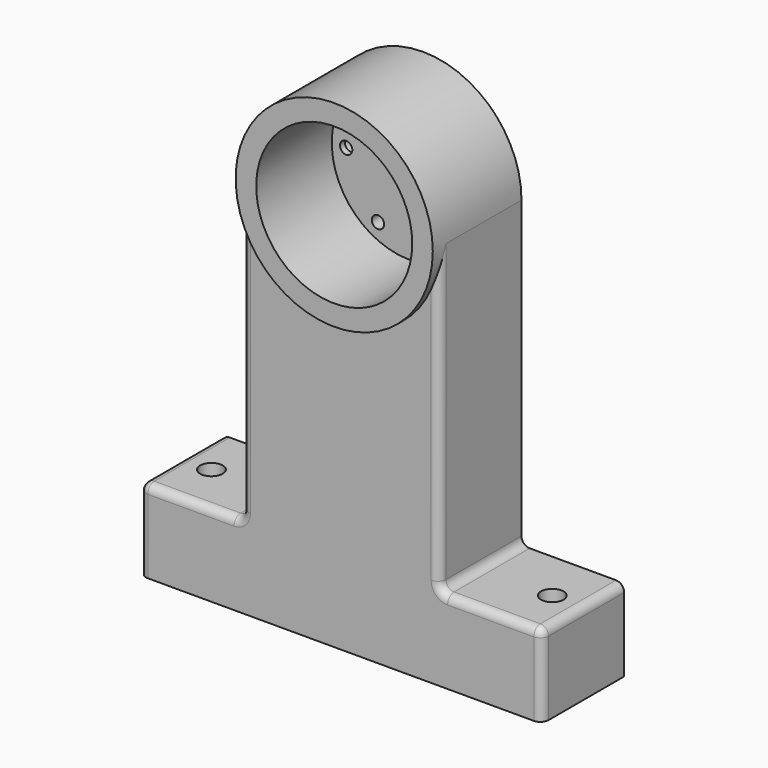
from build123d import *

# Parameters (mm, degrees)
F0_R          = 19
F0_R_2        = 1.5
F0_R_3        = 6.1
F1_DEPTH      = 4
F2_R          = 24
F2_R_2        = 19
F3_DEPTH      = 27
F5_DEPTH      = 25
F6_R          = 2.65
F7_DEPTH      = 2.5
F8_W          = 24
F8_H          = 54
F9_DEPTH      = 25
F10_W         = 25
F10_H         = 20
F11_DEPTH     = 25
F13_W         = 25
F13_H         = 20
F14_DEPTH     = 25
F15_R         = 2
F17_DEPTH     = 25
F18_DEPTH     = 25
F19_T1_DEPTH  = 25
F19_T3_DEPTH  = 21
F19_T5_DEPTH  = 23
F19_T7_DEPTH  = 21
F19_T12_DEPTH = 87
F19_S13_R     = 24
F19_T14_DEPTH = 45
F19_T18_DEPTH = 87
F19_S19_R     = 24
F19_T20_DEPTH = 45
F19_T22_ANGLE = 90
F19_T24_ANGLE = 90
F19_T26_ANGLE = 90
F19_T28_ANGLE = 90


# Not quite as in the source:
# - a fillet or chamfer that OpenCascade refuses, or shapes differently, is made with other operations: its cross-section is extruded or revolved along the edge and cut away or added


with BuildPart() as f1:
    # F0 (on Front) → F1 (new body)
    with BuildSketch(Plane.XZ):
        Circle(F0_R)
        with Locations((-7.75, -13.4233937587)):
            Circle(F0_R_2, mode=Mode.SUBTRACT)
        with Locations((7.75, -13.4233937587)):
            Circle(F0_R_2, mode=Mode.SUBTRACT)
        with Locations((-15.5, 0)):
            Circle(F0_R_2, mode=Mode.SUBTRACT)
        with Locations((-7.75, 13.4233937587)):
            Circle(F0_R_2, mode=Mode.SUBTRACT)
        with Locations((0, 7.1)):
            Circle(F0_R_3, mode=Mode.SUBTRACT)
        with BuildLine():
            ThreePointArc((14, 0), (15.5, 1.5), (17, 0))
            ThreePointArc((17, 0), (15.5, -1.5), (14, 0))
        make_face(mode=Mode.SUBTRACT)
        with Locations((7.75, 13.4233937587)):
            Circle(F0_R_2, mode=Mode.SUBTRACT)
    extrude(amount=F1_DEPTH)

    # F2 (on Front) → F3 (join)
    with BuildSketch(Plane.XZ):
        Circle(F2_R)
        Circle(F2_R_2, mode=Mode.SUBTRACT)
    extrude(amount=F3_DEPTH)

    # F4 (on face) → F5 (join)
    with BuildSketch(Plane(origin=(0, 0, 0), x_dir=(-1, 0, 0), z_dir=(0, 1, 0))):
        with BuildLine():
            Line((24, -40), (24, 0))
            ThreePointArc((24, 0), (0, -24), (-24, 0))
            Line((-24, 0), (-24, -40))
            Line((-24, -40), (0, -40))
            Line((0, -40), (24, -40))
        make_face()
    extrude(amount=-F5_DEPTH)

    # F6 (on face) → F7 (cut)
    with BuildSketch(Plane(origin=(0, 0, 0), x_dir=(-1, 0, 0), z_dir=(0, 1, 0))):
        with Locations((-7.75, 13.4233937587)):
            Circle(F6_R)
        with Locations((7.75, 13.4233937587)):
            Circle(F6_R)
        with Locations((-15.5, 0)):
            Circle(F6_R)
        with Locations((15.5, 0)):
            Circle(F6_R)
    extrude(amount=-F7_DEPTH, mode=Mode.SUBTRACT)

    # F8 (on face) → F9 (join, through all)
    with BuildSketch(Plane.XZ.offset(25)):
        with Locations((12, -67)):
            Rectangle(F8_W, F8_H)
        with Locations((-12, -67)):
            Rectangle(F8_W, F8_H)
    extrude(amount=-F9_DEPTH)

    # F10 (on face) → F11 (join)
    with BuildSketch(Plane.YZ.offset(24)):
        with Locations((-12.5, -84)):
            Rectangle(F10_W, F10_H)
    extrude(amount=F11_DEPTH)

    # F13 (on face) → F14 (join)
    with BuildSketch(Plane(origin=(-24, 0, 0), x_dir=(0, -1, 0), z_dir=(-1, 0, 0))):
        with Locations((12.5, -84)):
            Rectangle(F13_W, F13_H)
    extrude(amount=F14_DEPTH)

    # F15
    f15_edges = [f1.edges().sort_by_distance(p)[0] for p in [
        (49, -12.5, -74),
        (-49, -12.5, -74),
    ]]
    fillet(f15_edges, radius=F15_R)

    # F16 (on face) → F17 (cut)
    with BuildSketch(Plane(origin=(0, 0, -94), x_dir=(1, 0, 0), z_dir=(0, 0, -1))):
        with BuildLine():
            ThreePointArc((-38.75, 12.5), (-41.5, 15.25), (-44.25, 12.5))
            Line((-44.25, 12.5), (-38.75, 12.5))
        make_face()
        with BuildLine():
            Line((-38.75, 12.5), (-44.25, 12.5))
            ThreePointArc((-44.25, 12.5), (-41.5, 9.75), (-38.75, 12.5))
        make_face()
    extrude(amount=-F17_DEPTH, mode=Mode.SUBTRACT)

    # F12 (on face) → F18 (cut)
    with BuildSketch(Plane.XY.offset(-74)):
        with BuildLine():
            ThreePointArc((38.75, -12.5), (41.5, -15.25), (44.25, -12.5))
            Line((44.25, -12.5), (38.75, -12.5))
        make_face()
        with BuildLine():
            Line((38.75, -12.5), (44.25, -12.5))
            ThreePointArc((44.25, -12.5), (41.5, -9.75), (38.75, -12.5))
        make_face()
    extrude(amount=-F18_DEPTH, mode=Mode.SUBTRACT)

    # F19: fillet of radius 2 on 10 edges, made by hand

    # F19_s2 → F19_t1 (join)
    with BuildSketch(Plane.XZ):
        with BuildLine():
            ThreePointArc((24, -72), (24.5857864376, -73.4142135624), (26, -74))
            Line((26, -74), (24, -74))
            Line((24, -74), (24, -72))
        make_face()
        with BuildLine():
            ThreePointArc((-26, -74), (-24.5857864376, -73.4142135624), (-24, -72))
            Line((-24, -72), (-24, -74))
            Line((-24, -74), (-26, -74))
        make_face()
    extrude(amount=F19_T1_DEPTH)

    # F19_s4 → F19_t3 (cut)
    with BuildSketch(Plane.YZ.offset(-47)):
        with BuildLine():
            ThreePointArc((-23, -74), (-24.4142135624, -74.5857864376), (-25, -76))
            Line((-25, -76), (-25, -74))
            Line((-25, -74), (-23, -74))
        make_face()
    extrude(amount=F19_T3_DEPTH, mode=Mode.SUBTRACT)

    # F19_s6 → F19_t5 (cut)
    with BuildSketch(Plane.XY.offset(-99)):
        with BuildLine():
            ThreePointArc((-49, -23), (-48.4142135624, -24.4142135624), (-47, -25))
            Line((-47, -25), (-49, -25))
            Line((-49, -25), (-49, -23))
        make_face()
        with BuildLine():
            ThreePointArc((49, -23), (48.4142135624, -24.4142135624), (47, -25))
            Line((47, -25), (49, -25))
            Line((49, -25), (49, -23))
        make_face()
    extrude(amount=F19_T5_DEPTH, mode=Mode.SUBTRACT)

    # F19_s8 → F19_t7 (cut)
    with BuildSketch(Plane.YZ.offset(26)):
        with BuildLine():
            ThreePointArc((-23, -74), (-24.4142135624, -74.5857864376), (-25, -76))
            Line((-25, -76), (-25, -74))
            Line((-25, -74), (-23, -74))
        make_face()
    extrude(amount=F19_T7_DEPTH, mode=Mode.SUBTRACT)


with BuildPart() as f19_tool10:
    # F19_s11 → F19_t12 (new body)
    with BuildSketch(Plane.XY.offset(15)):
        with BuildLine():
            ThreePointArc((24, -23), (23.4142135624, -24.4142135624), (22, -25))
            Line((22, -25), (24, -25))
            Line((24, -25), (24, -23))
        make_face()
    extrude(amount=-F19_T12_DEPTH)

    # F19_s13 → F19_t14 (cut, symmetric)
    with BuildSketch(Plane.XZ.offset(24)):
        Circle(F19_S13_R)
    extrude(amount=F19_T14_DEPTH, both=True, mode=Mode.SUBTRACT)


with BuildPart() as f1_1:
    add(f1.part)

    # F19_t9: cut F19_tool10
    add(f19_tool10.part, mode=Mode.SUBTRACT)


with BuildPart() as f19_tool16:
    # F19_s17 → F19_t18 (new body)
    with BuildSketch(Plane.XY.offset(-72)):
        with BuildLine():
            ThreePointArc((-24, -23), (-23.4142135624, -24.4142135624), (-22, -25))
            Line((-22, -25), (-24, -25))
            Line((-24, -25), (-24, -23))
        make_face()
    extrude(amount=F19_T18_DEPTH)

    # F19_s19 → F19_t20 (cut, symmetric)
    with BuildSketch(Plane.XZ.offset(24)):
        Circle(F19_S19_R)
    extrude(amount=F19_T20_DEPTH, both=True, mode=Mode.SUBTRACT)


with BuildPart() as f1_2:
    add(f1_1.part)

    # F19_t15: cut F19_tool16
    add(f19_tool16.part, mode=Mode.SUBTRACT)

    # F19_s21 → F19_t22 (revolve, cut)
    with BuildSketch(Plane.XY.offset(-76)):
        with BuildLine():
            ThreePointArc((-49, -23), (-48.4142135624, -24.4142135624), (-47, -25))
            Line((-47, -25), (-49, -25))
            Line((-49, -25), (-49, -23))
        make_face()
    revolve(axis=Axis((-47, -25, -76), (0, 1, 0)), revolution_arc=F19_T22_ANGLE, mode=Mode.SUBTRACT)

    # F19_s23 → F19_t24 (revolve, cut)
    with BuildSketch(Plane.YZ.offset(47)):
        with BuildLine():
            ThreePointArc((-23, -74), (-24.4142135624, -74.5857864376), (-25, -76))
            Line((-25, -76), (-25, -74))
            Line((-25, -74), (-23, -74))
        make_face()
    revolve(axis=Axis((47, -25, -76), (0, 1, 0)), revolution_arc=F19_T24_ANGLE, mode=Mode.SUBTRACT)

    # F19_s25 → F19_t26 (revolve, cut)
    with BuildSketch(Plane.XY.offset(-72)):
        with BuildLine():
            ThreePointArc((22, -25), (23.4142135624, -24.4142135624), (24, -23))
            Line((24, -23), (24, -25))
            Line((24, -25), (22, -25))
        make_face()
    revolve(axis=Axis((26, -25, -72), (0, -1, 0)), revolution_arc=F19_T26_ANGLE, mode=Mode.SUBTRACT)

    # F19_s27 → F19_t28 (revolve, cut)
    with BuildSketch(Plane.YZ.offset(-26)):
        with BuildLine():
            ThreePointArc((-23, -74), (-24.4142135624, -74.5857864376), (-25, -76))
            Line((-25, -76), (-25, -74))
            Line((-25, -74), (-23, -74))
        make_face()
    revolve(axis=Axis((-26, -25, -72), (0, -1, 0)), revolution_arc=F19_T28_ANGLE, mode=Mode.SUBTRACT)


solid = f1_2.part
